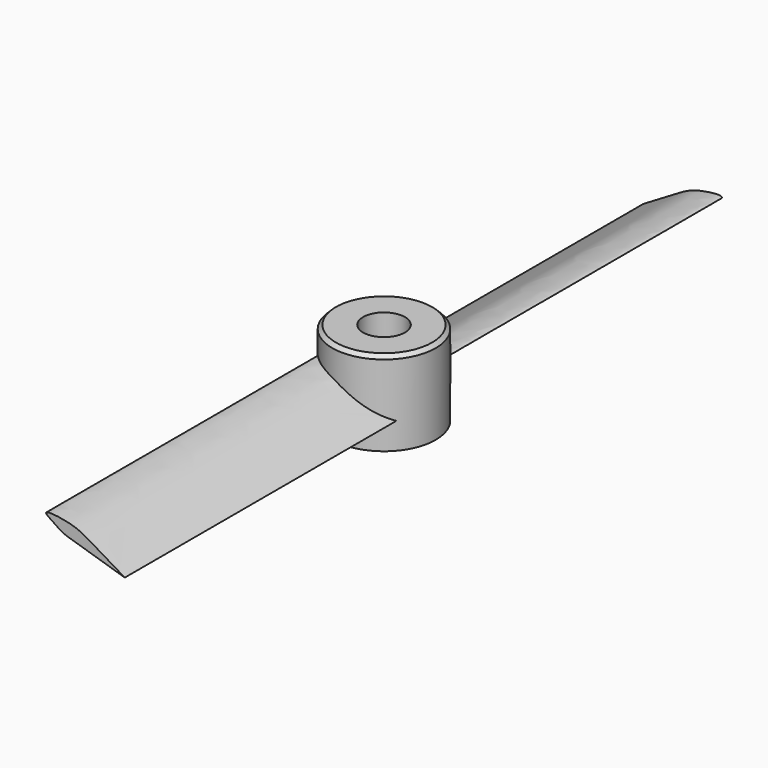
from build123d import *

# Parameters (mm, degrees)
F0_R     = 7.05
F0_R_2   = 2.85
F1_DEPTH = 11.5
F3_DEPTH = 50.8
F4_R     = 5
F6_DEPTH = 50.8
F7_R     = 5
F8_DEPTH = 25
F9_SIZE  = 0.5


# Not quite as in the source:
# - a feature names something its author has since deleted; it is built from what else it names


with BuildPart() as f1:
    # F0 (on Top) → F1 (new body)
    with BuildSketch(Plane.XY):
        Circle(F0_R)
        Circle(F0_R_2, mode=Mode.SUBTRACT)
        Circle(F0_R_2)
    extrude(amount=F1_DEPTH)

    # F2 (on Front) → F3 (join)
    with BuildSketch(Plane.XZ):
        with BuildLine():
            add(Edge.make_bspline(
                [(-3.0868715491, 6.1726554698), (-4.257758818, 7.0278775794), (-6.7334588292, 8.3125277988), (-2.2069270317, 7.8156179057), (-0.1331950402, 6.9264711716), (2.6616102749, 5.1687815765), (4.451992816, 4.1126824333), (5.3511540891, 3.588018488)],
                knots=[0, 0, 0, 0, 0.1977876363, 0.3919769243, 0.5835513721, 0.7917756861, 1, 1, 1, 1], degree=3))
            Line((-3.0868715491, 6.1726554698), (5.3511540891, 3.588018488))
        make_face()
    extrude(amount=F3_DEPTH)

    # F4
    f4_edges = [f1.edges().sort_by_distance(p)[0] for p in [
        (-3.086872, -28.569137, 6.172655),
    ]]
    fillet(f4_edges, radius=F4_R)

    # F5 (on Front) → F6 (join)
    with BuildSketch(Plane.XZ):
        with BuildLine():
            Line((-5.3514227233, 3.587880028), (3.086602915, 6.1725170098))
            add(Edge.make_bspline(
                [(3.086602915, 6.1725170098), (4.2574901838, 7.0277391194), (6.733190195, 8.3123893387), (2.2066583976, 7.8154794457), (0.1329264061, 6.9263327116), (-2.661878909, 5.1686431165), (-4.4522614501, 4.1125439733), (-5.3514227233, 3.587880028)],
                knots=[0, 0, 0, 0, 0.1977876363, 0.3919769243, 0.5835513721, 0.7917756861, 1, 1, 1, 1], degree=3))
        make_face()
    extrude(amount=-F6_DEPTH)

    # F7
    f7_edges = [f1.edges().sort_by_distance(p)[0] for p in [
        (3.086603, 28.569203, 6.172517),
    ]]
    fillet(f7_edges, radius=F7_R)

    # F0 (on Top) → F8 (cut)
    with BuildSketch(Plane.XY):
        Circle(F0_R_2)
    extrude(amount=F8_DEPTH, mode=Mode.SUBTRACT)

    # F9
    f9_edges = [f1.edges().sort_by_distance(p)[0] for p in [
        (-7.05, 0, 11.5),
    ]]
    chamfer(f9_edges, length=F9_SIZE)


solid = f1.part
